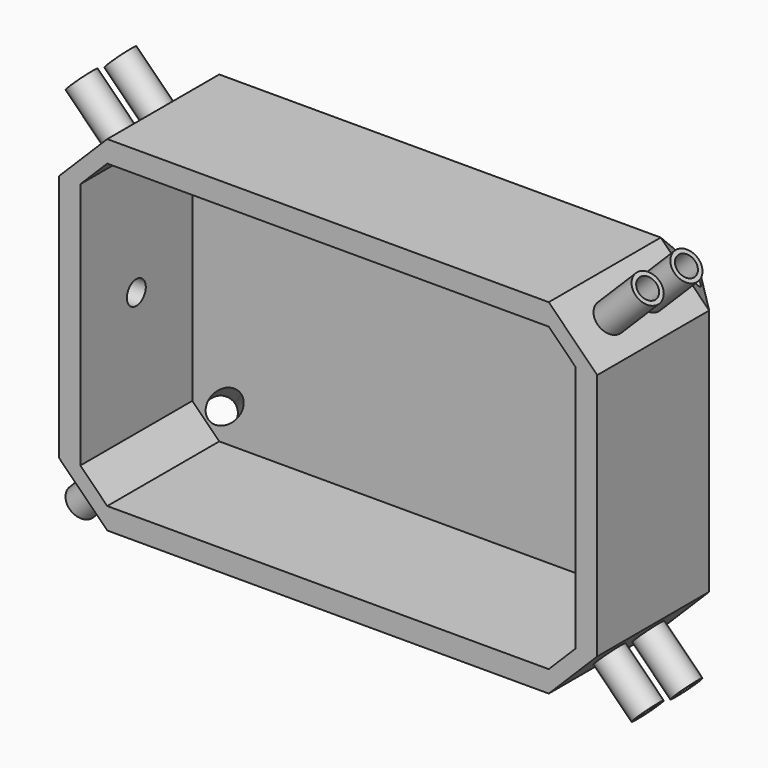
from build123d import *

# Parameters (mm, degrees)
F0_W      = 50
F0_H      = 32
F1_DEPTH  = 24
F2_SIZE   = 4.5
F3_W      = 64.6181842312
F3_H      = 72.6516954601
F4_DEPTH  = 6.5
F6_DEPTH  = 13
F7_R      = 1.4
F8_DEPTH  = 5
F9_R      = 1.4
F10_DEPTH = 5
F11_R     = 1.4
F12_DEPTH = 5
F13_R     = 1.4
F14_DEPTH = 5
F15_R     = 1
F16_DEPTH = 5
F17_R     = 1
F18_DEPTH = 5
F19_R     = 1
F20_DEPTH = 5
F21_R     = 1
F22_DEPTH = 5
F23_R     = 1.1
F24_DEPTH = 25.4
F25_R     = 1.25
F26_DEPTH = 25.4
F27_R     = 1.25
F28_DEPTH = 25.4
F30_DEPTH = 25.4
F32_DEPTH = 25.4


# Not quite as in the source:
# - a feature names something its author has since deleted; it is built from what else it names


with BuildPart() as f1:
    # F0 (on Front) → F1 (new body)
    with BuildSketch(Plane.XZ):
        with Locations((25, 16)):
            Rectangle(F0_W, F0_H)
    extrude(amount=F1_DEPTH)

    # F2
    f2_edges = [f1.edges().sort_by_distance(p)[0] for p in [
        (50, -12, 0),
        (50, -12, 32),
        (50, 0, 16),
        (50, -24, 16),
        (0, -12, 32),
        (25, 0, 32),
        (25, -24, 32),
        (0, -12, 0),
        (0, 0, 16),
        (0, -24, 16),
        (25, 0, 0),
        (25, -24, 0),
    ]]
    chamfer(f2_edges, length=F2_SIZE)

    # F3 (on face) → F4 (cut)
    with BuildSketch(Plane.XZ.offset(24)):
        with Locations((22.701323498, 16.0673912615)):
            Rectangle(F3_W, F3_H)
    extrude(amount=-F4_DEPTH, mode=Mode.SUBTRACT)

    # F5 (on face) → F6 (cut)
    with BuildSketch(Plane.XZ.offset(17.5)):
        Polygon((4.5, 30), (2, 27.5), (2, 4.5), (4.5, 2), (45.5, 2), (48, 4.5), (48, 27.5), (45.5, 30), align=None)
    extrude(amount=-F6_DEPTH, mode=Mode.SUBTRACT)

    # F7 (on face) → F8 (join)
    with BuildSketch(Plane(origin=(38.75, 0, 38.75), x_dir=(0, 1, 0), z_dir=(0.7071067812, 0, 0.7071067812))):
        with Locations((-13.25, -12.7279220614)):
            Circle(F7_R)
        with Locations((-8.75, -12.7279220614)):
            Circle(F7_R)
    extrude(amount=F8_DEPTH)

    # F9 (on face) → F10 (join)
    with BuildSketch(Plane(origin=(22.75, 0, -22.75), x_dir=(0, 1, 0), z_dir=(0.7071067812, 0, -0.7071067812))):
        with Locations((-13.25, 35.3553390593)):
            Circle(F9_R)
        with Locations((-8.75, 35.3553390593)):
            Circle(F9_R)
    extrude(amount=F10_DEPTH)

    # F11 (on face) → F12 (join)
    with BuildSketch(Plane(origin=(2.25, 0, 2.25), x_dir=(0, -1, 0), z_dir=(-0.7071067812, 0, -0.7071067812))):
        with Locations((13.25, 0)):
            Circle(F11_R)
        with Locations((8.75, 0)):
            Circle(F11_R)
    extrude(amount=F12_DEPTH)

    # F13 (on face) → F14 (join)
    with BuildSketch(Plane(origin=(-13.75, 0, 13.75), x_dir=(0, -1, 0), z_dir=(-0.7071067812, 0, 0.7071067812))):
        with Locations((8.75, 22.6343975133)):
            Circle(F13_R)
        with Locations((13.25, 22.6343975133)):
            Circle(F13_R)
    extrude(amount=F14_DEPTH)

    # F15 (on face) → F16 (cut)
    with BuildSketch(Plane(origin=(42.2855339059, 0, 42.2855339059), x_dir=(0, 1, 0), z_dir=(0.7071067812, 0, 0.7071067812))):
        with Locations((-13.25, -12.7279220614)):
            Circle(F15_R)
        with Locations((-8.75, -12.7279220614)):
            Circle(F15_R)
    extrude(amount=-F16_DEPTH, mode=Mode.SUBTRACT)

    # F17 (on face) → F18 (cut)
    with BuildSketch(Plane(origin=(26.2855339059, 0, -26.2855339059), x_dir=(0, 1, 0), z_dir=(0.7071067812, 0, -0.7071067812))):
        with Locations((-13.25, 35.3553390593)):
            Circle(F17_R)
        with Locations((-8.75, 35.3553390593)):
            Circle(F17_R)
    extrude(amount=-F18_DEPTH, mode=Mode.SUBTRACT)

    # F19 (on face) → F20 (cut)
    with BuildSketch(Plane(origin=(-1.2855339059, 0, -1.2855339059), x_dir=(0, -1, 0), z_dir=(-0.7071067812, 0, -0.7071067812))):
        with Locations((13.25, 0)):
            Circle(F19_R)
        with Locations((8.75, 0)):
            Circle(F19_R)
    extrude(amount=-F20_DEPTH, mode=Mode.SUBTRACT)

    # F21 (on face) → F22 (cut)
    with BuildSketch(Plane(origin=(-17.2855339059, 0, 17.2855339059), x_dir=(0, -1, 0), z_dir=(-0.7071067812, 0, 0.7071067812))):
        with Locations((8.75, 22.6343975133)):
            Circle(F21_R)
        with Locations((13.25, 22.6343975133)):
            Circle(F21_R)
    extrude(amount=-F22_DEPTH, mode=Mode.SUBTRACT)

    # F23 (on face) → F24 (cut)
    with BuildSketch(Plane(origin=(0, 0, 0), x_dir=(0, -1, 0), z_dir=(-1, 0, 0))):
        with Locations((11, 16.0062)):
            Circle(F23_R)
    extrude(amount=-F24_DEPTH, mode=Mode.SUBTRACT)

    # F25 (on face) → F26 (cut)
    with BuildSketch(Plane(origin=(24.3333333333, 24.3333333333, 24.3333333333), x_dir=(-0.4082482905, 0.8164965809, -0.4082482905), z_dir=(0.5773502692, 0.5773502692, 0.5773502692))):
        with Locations((-33.0634771251, -12.7279220614)):
            Circle(F25_R)
    extrude(amount=-F26_DEPTH, mode=Mode.SUBTRACT)

    # F27 (on face) → F28 (cut)
    with BuildSketch(Plane(origin=(13.6666666667, 13.6666666667, -13.6666666667), x_dir=(-0.4082482905, 0.8164965809, 0.4082482905), z_dir=(0.5773502692, 0.5773502692, -0.5773502692))):
        with Locations((-19.7495318303, 35.3553390593)):
            Circle(F27_R)
    extrude(amount=-F28_DEPTH, mode=Mode.SUBTRACT)

    # F29 (on face) → F30 (cut)
    with BuildSketch(Plane(origin=(-7.6666666667, 7.6666666667, 7.6666666667), x_dir=(-0.8164965809, -0.4082482905, -0.4082482905), z_dir=(-0.5773502692, 0.5773502692, 0.5773502692))):
        with BuildLine():
            ThreePointArc((-12.8330958098, 23.027260035), (-14.5406275645, 22.5697282803), (-14.0830958098, 20.8621965255))
            Line((-14.0830958098, 20.8621965255), (-12.8330958098, 23.027260035))
        make_face()
        with BuildLine():
            Line((-12.8330958098, 23.027260035), (-14.0830958098, 20.8621965255))
            ThreePointArc((-14.0830958098, 20.8621965255), (-12.8330958098, 20.8621965255), (-12.2080958098, 21.9447282803))
            ThreePointArc((-12.2080958098, 21.9447282803), (-12.3755640551, 22.5697282803), (-12.8330958098, 23.027260035))
        make_face()
    extrude(amount=-F30_DEPTH, mode=Mode.SUBTRACT)

    # F31 (on face) → F32 (cut)
    with BuildSketch(Plane(origin=(3, -3, 3), x_dir=(-0.8164965809, -0.4082482905, 0.4082482905), z_dir=(-0.5773502692, 0.5773502692, -0.5773502692))):
        with BuildLine():
            ThreePointArc((1.0435586535, 0.3575669008), (0.4185586535, 1.4400986556), (-0.8314413465, 1.4400986556))
            Line((-0.8314413465, 1.4400986556), (0.4185586535, -0.7249648539))
            ThreePointArc((0.4185586535, -0.7249648539), (0.8760904083, -0.2674330992), (1.0435586535, 0.3575669008))
        make_face()
        with BuildLine():
            Line((0.4185586535, -0.7249648539), (-0.8314413465, 1.4400986556))
            ThreePointArc((-0.8314413465, 1.4400986556), (-1.2889731012, -0.2674330992), (0.4185586535, -0.7249648539))
        make_face()
    extrude(amount=-F32_DEPTH, mode=Mode.SUBTRACT)


solid = f1.part
